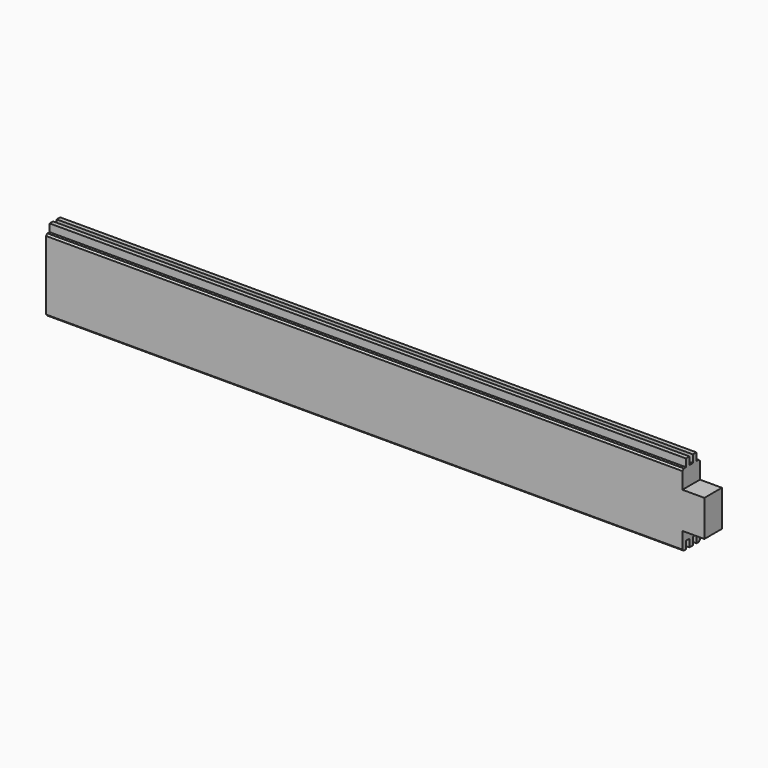
from build123d import *

# Parameters (mm, degrees)
F1_W     = 40
F1_H     = 33
F3_DEPTH = 600
F2_W     = 80
F2_H     = 100
F4_DEPTH = 25


with BuildPart() as f3:
    # F1 (on Right) → F3 (new body, symmetric)
    with BuildSketch(Plane.YZ):
        Polygon((20, 33), (20, 63), (17, 66), (12, 66), (12, 80), (4, 80), (4, 66), (-4, 66), (-4, 80), (-12, 80), (-12, 66), (-17, 66), (-20, 63), (-20, 33), align=None)
        with Locations((0, 16.5)):
            Rectangle(F1_W, F1_H)
        with Locations((0, -16.5)):
            Rectangle(F1_W, F1_H)
        Polygon((20, -63), (20, -33), (-20, -33), (-20, -63), (-17, -66), (-12, -66), (-12, -52), (-4, -52), (-4, -66), (4, -66), (4, -52), (12, -52), (12, -66), (17, -66), align=None)
    extrude(amount=F3_DEPTH, both=True)

    # F2 (on Front) → F4 (cut, symmetric)
    with BuildSketch(Plane.XZ):
        with Locations((600, 83)):
            Rectangle(F2_W, F2_H)
        with Locations((600, -83)):
            Rectangle(F2_W, F2_H)
    extrude(amount=F4_DEPTH, both=True, mode=Mode.SUBTRACT)


solid = f3.part
